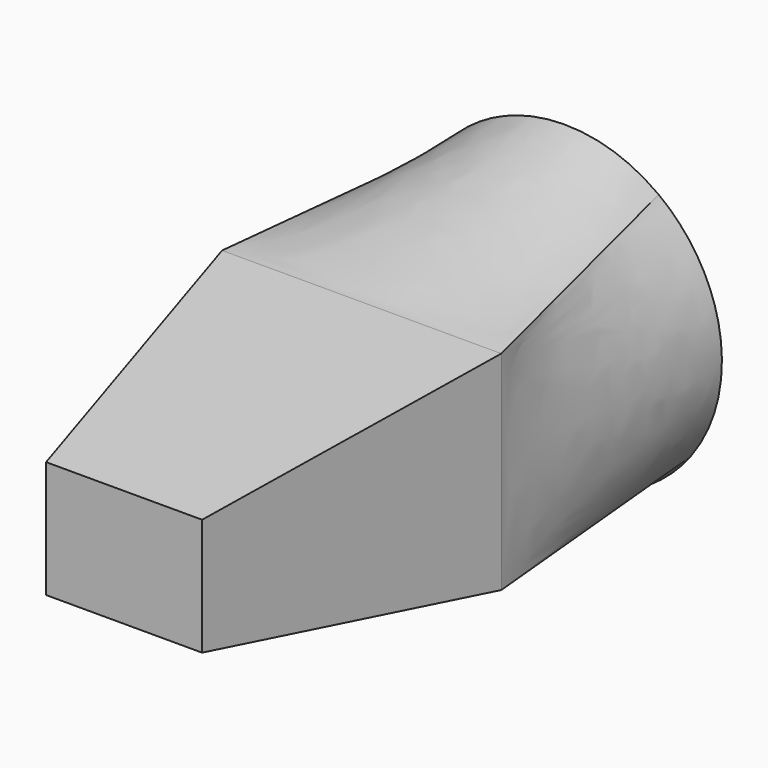
from build123d import *

# Parameters (mm, degrees)
F2_W      = 27.9399994761
F2_H      = 20.8280012012
F3_FACE_W = 27.9399994761
F3_FACE_H = 20.8280012012
F5_W      = 15.6096592546
F5_H      = 11.7110861465


# Not quite as in the source:
# - the arcs of a loft's sections are written as splines that run evenly, so that the points pair up as in the source's solid


with BuildPart() as f3:
    # F0 (on Front) → F3 section 0
    with BuildSketch(Plane.XZ):
        with BuildLine():
            add(Edge.make_bspline(
                [(-12.6098715409, 9.4000867761), (-13.8403400225, 7.7494584513), (-14.7421231636, 5.8548204804), (-15.7523962289, 1.8630972263), (-15.8604886539, -0.2324174842), (-15.2662929053, -4.3069036624), (-14.5642385224, -6.2842719937), (-12.4560348761, -9.8212175107), (-11.050715101, -11.3794030593), (-9.4000867761, -12.6098715409)],
                knots=[0, 0, 0, 0, 0.25, 0.25, 0.5, 0.5, 0.75, 0.75, 1, 1, 1, 1], degree=3))
            add(Edge.make_bspline(
                [(-9.4000867761, -12.6098715409), (-7.7494584513, -13.8403400225), (-5.8548204804, -14.7421231636), (-1.8630972263, -15.7523962289), (0.2324174842, -15.8604886539), (4.3069036624, -15.2662929053), (6.2842719937, -14.5642385224), (9.8212175107, -12.4560348761), (11.3794030593, -11.050715101), (12.6098715409, -9.4000867761)],
                knots=[0, 0, 0, 0, 0.25, 0.25, 0.5, 0.5, 0.75, 0.75, 1, 1, 1, 1], degree=3))
            add(Edge.make_bspline(
                [(12.6098715409, -9.4000867761), (13.8403400225, -7.7494584513), (14.7421231636, -5.8548204804), (15.7523962289, -1.8630972263), (15.8604886539, 0.2324174842), (15.2662929053, 4.3069036624), (14.5642385224, 6.2842719937), (12.4560348761, 9.8212175107), (11.050715101, 11.3794030593), (9.4000867761, 12.6098715409)],
                knots=[0, 0, 0, 0, 0.25, 0.25, 0.5, 0.5, 0.75, 0.75, 1, 1, 1, 1], degree=3))
            add(Edge.make_bspline(
                [(9.4000867761, 12.6098715409), (7.7494584513, 13.8403400225), (5.8548204804, 14.7421231636), (1.8630972263, 15.7523962289), (-0.2324174842, 15.8604886539), (-4.3069036624, 15.2662929053), (-6.2842719937, 14.5642385224), (-9.8212175107, 12.4560348761), (-11.3794030593, 11.050715101), (-12.6098715409, 9.4000867761)],
                knots=[0, 0, 0, 0, 0.25, 0.25, 0.5, 0.5, 0.75, 0.75, 1, 1, 1, 1], degree=3))
        make_face()
    # F2 (on offset) → F3 section 1
    with BuildSketch(Plane.XZ.offset(25.4)):
        Rectangle(F2_W, F2_H)
    loft(ruled=True)

    # F3_face (on face) → F6 section 0
    with BuildSketch(Plane.XZ.offset(25.4)):
        Rectangle(F3_FACE_W, F3_FACE_H)
    # F5 (on offset) → F6 section 1
    with BuildSketch(Plane.XZ.offset(55.118)):
        Rectangle(F5_W, F5_H)
    loft()


solid = f3.part
